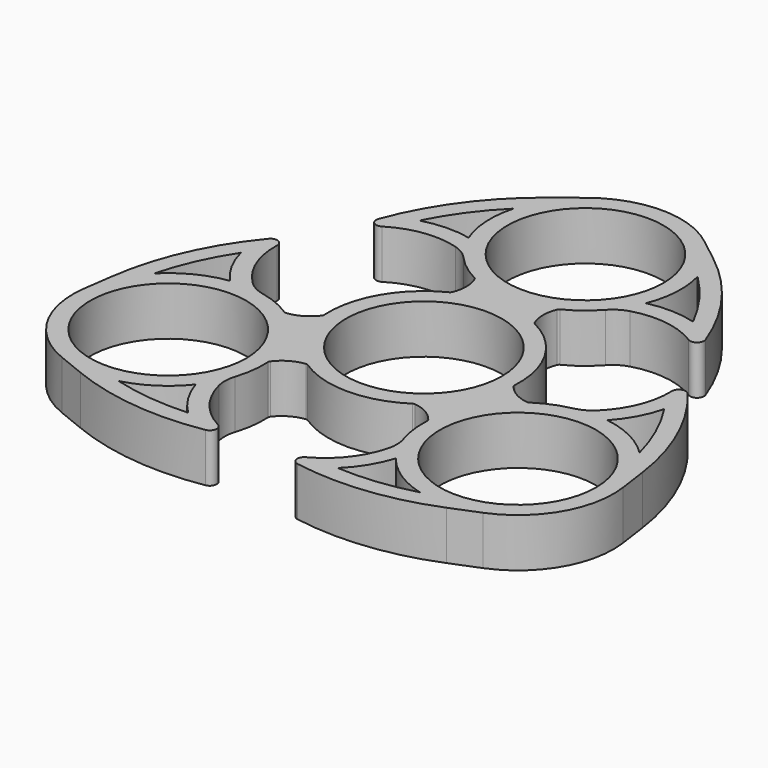
from build123d import *

# Parameters (mm, degrees)
F0_R     = 11.2
F1_DEPTH = 7
F3_R     = 1
F4_R     = 5
F5_R     = 0.5
F6_R     = 1952.4287438443
F7_COUNT = 3


# Not quite as in the source:
# - a feature names something its author has since deleted; it is built from what else it names


with BuildPart() as f1:
    # F0 (on Top) → F1 (new body)
    with BuildSketch(Plane.XY):
        with BuildLine():
            ThreePointArc((-6, 16.6837505709), (-5.5170914007, 14.5), (-6, 12.3162494291))
            ThreePointArc((-6, 12.3162494291), (0, -13.7), (6, 12.3162494291))
            ThreePointArc((6, 12.3162494291), (5.5170914007, 14.5), (6, 16.6837505709))
            ThreePointArc((6, 16.6837505709), (8.6909924163, 18.4095962862), (10.9087481118, 20.7121043302))
            ThreePointArc((10.9087481118, 20.7121043302), (18.1728004264, 21.5386604601), (24.5200451463, 17.9106947035))
            ThreePointArc((24.5200451463, 17.9106947035), (18.9966635049, 29.6635307849), (9.6725196457, 38.7021834503))
            ThreePointArc((9.6725196457, 38.7021834503), (-11.1613035419, 36.9445140346), (-6, 16.6837505709))
        make_face()
        Circle(F0_R, mode=Mode.SUBTRACT)
        with Locations((0, 29)):
            Circle(F0_R, mode=Mode.SUBTRACT)
        with BuildLine():
            ThreePointArc((13.2182511873, 32.6010881063), (16.7973161482, 28.4394734973), (19.6512198892, 23.7507662571))
            ThreePointArc((19.6512198892, 23.7507662571), (16.2043181529, 24.2743066369), (12.733437995, 23.9453430554))
            ThreePointArc((12.733437995, 23.9453430554), (13.6785607229, 28.2338560515), (13.2182511873, 32.6010881063))
        make_face(mode=Mode.SUBTRACT)
    extrude(amount=F1_DEPTH)

    # F3
    f3_edges = [f1.edges().sort_by_distance(p)[0] for p in [
        (24.520045, 17.910695, 3.5),
    ]]
    fillet(f3_edges, radius=F3_R)

    # F4
    f4_edges = [f1.edges().sort_by_distance(p)[0] for p in [
        (10.908748, 20.712104, 3.5),
    ]]
    fillet(f4_edges, radius=F4_R)

    # F5
    f5_edges = [f1.edges().sort_by_distance(p)[0] for p in [
        (-6, 16.683751, 3.5),
        (-6, 12.316249, 3.5),
        (6, 16.683751, 3.5),
        (6, 12.316249, 3.5),
    ]]
    fillet(f5_edges, radius=F5_R)

    # F6
    f6_edges = [f1.edges().sort_by_distance(p)[0] for p in [
        (9.67252, 38.702183, 3.5),
    ]]
    fillet(f6_edges, radius=F6_R)

    # F7: F1 ×3 about axis
    f7_axis = Axis((0, 0, 12.0743541047), (0, 0, 1))


with BuildPart() as f1_1:
    add(f1.part)
    for i in range(1, F7_COUNT):
        add(f1.part.rotate(f7_axis, i * 360 / F7_COUNT))

    # F8: F1 across plane


with BuildPart() as f1_2:
    add(f1_1.part)
    add(f1_1.part.mirror(Plane.YZ))


solid = f1_2.part
